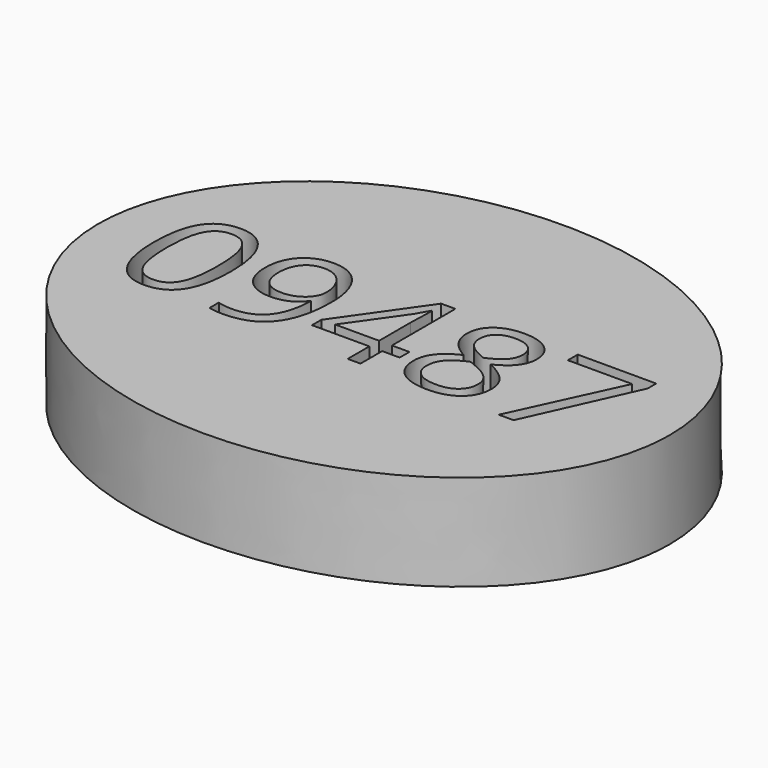
from build123d import *

# Parameters (mm, degrees)
F1_DEPTH     = 25.4
F2_TEXT_SIZE = 43.6701876525
F3_DEPTH     = 25.4


# Not quite as in the source:
# - Text() gives the source's letters only with a copy of the font that has no kerning and outlines rounded to 1/6400 em; it was checked with that copy


with BuildPart() as f1:
    # F0 (on Top) → F1 (new body)
    with BuildSketch(Plane.XY):
        with BuildLine():
            add(Edge.make_bspline(
                [(75.5536705256, -2.289499389), (75.5536705256, 100.8530168189), (-37.7768352628, 49.281758715), (-151.1073410511, -2.289499389), (-37.7768352628, -53.860757493), (75.5536705256, -105.432015597), (75.5536705256, -2.289499389)],
                knots=[0, 0, 0, 2.0943951024, 2.0943951024, 4.1887902048, 4.1887902048, 6.2831853072, 6.2831853072, 6.2831853072], degree=2, weights=[1, 0.5, 1, 0.5, 1, 0.5, 1]))
        make_face()
    extrude(amount=F1_DEPTH)

    # F2 (on face) → F3 (cut)
    with BuildSketch(Plane.XY.offset(25.4)):
        with Locations((-63.6482387781, -17.2476070002)):
            Text('09487', F2_TEXT_SIZE, font='Open Sans', text_align=(TextAlign.LEFT, TextAlign.BOTTOM))
    extrude(amount=-F3_DEPTH, mode=Mode.SUBTRACT)


solid = f1.part
